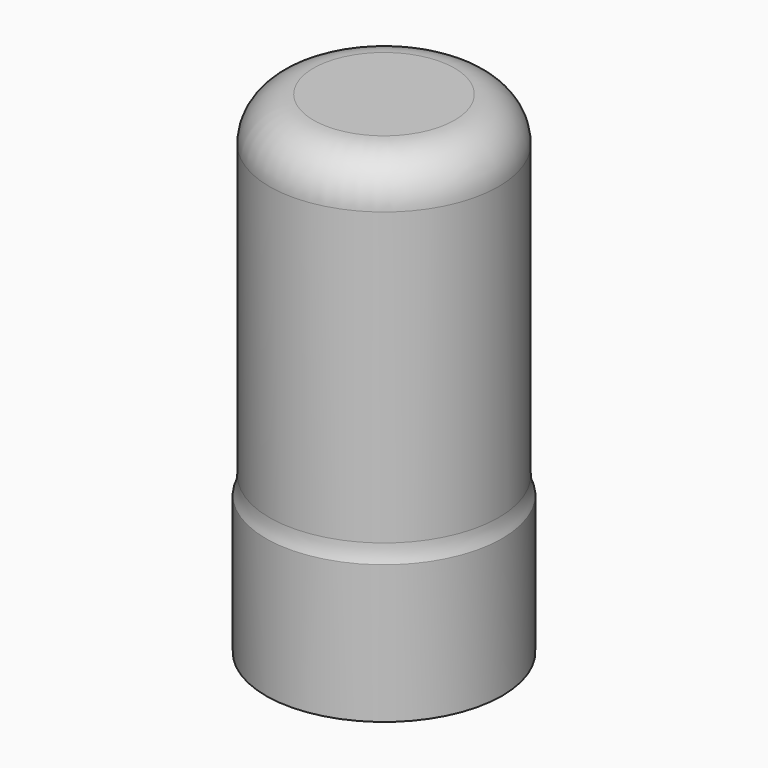
from build123d import *

# Parameters (mm, degrees)
F0_R     = 3.4036
F1_DEPTH = 3.9878
F2_R     = 3.302
F3_DEPTH = 10.16


# Not quite as in the source:
# - a fillet or chamfer that OpenCascade refuses, or shapes differently, is made with other operations: its cross-section is extruded or revolved along the edge and cut away or added


with BuildPart() as f1:
    # F0 (on Top) → F1 (new body)
    with BuildSketch(Plane.XY):
        Circle(F0_R)
    extrude(amount=F1_DEPTH)

    # F2 (on face) → F3 (join)
    with BuildSketch(Plane.XY.offset(3.9878)):
        Circle(F2_R)
    extrude(amount=F3_DEPTH)

    # F4: fillet of radius 1.27 on 2 edges, made by hand

    # F4_s1 → F4_t2 (revolve)
    with BuildSketch(Plane.XZ):
        with BuildLine():
            ThreePointArc((3.4036, 3.9878), (3.3276592107, 4.2315363157), (3.302, 4.4855363157))
            Line((3.302, 4.4855363157), (3.302, 3.9878))
            Line((3.302, 3.9878), (3.4036, 3.9878))
        make_face()
    revolve(axis=Axis((0, 0, 3.9878), (0, 0, 1)))

    # F4_s3 → F4_t4 (revolve, cut)
    with BuildSketch(Plane.XZ):
        with BuildLine():
            ThreePointArc((3.302, 12.8778), (2.9300256121, 13.7758256121), (2.032, 14.1478))
            Line((2.032, 14.1478), (3.302, 14.1478))
            Line((3.302, 14.1478), (3.302, 12.8778))
        make_face()
    revolve(axis=Axis((0, 0, 14.1478), (0, 0, 1)), mode=Mode.SUBTRACT)


solid = f1.part
